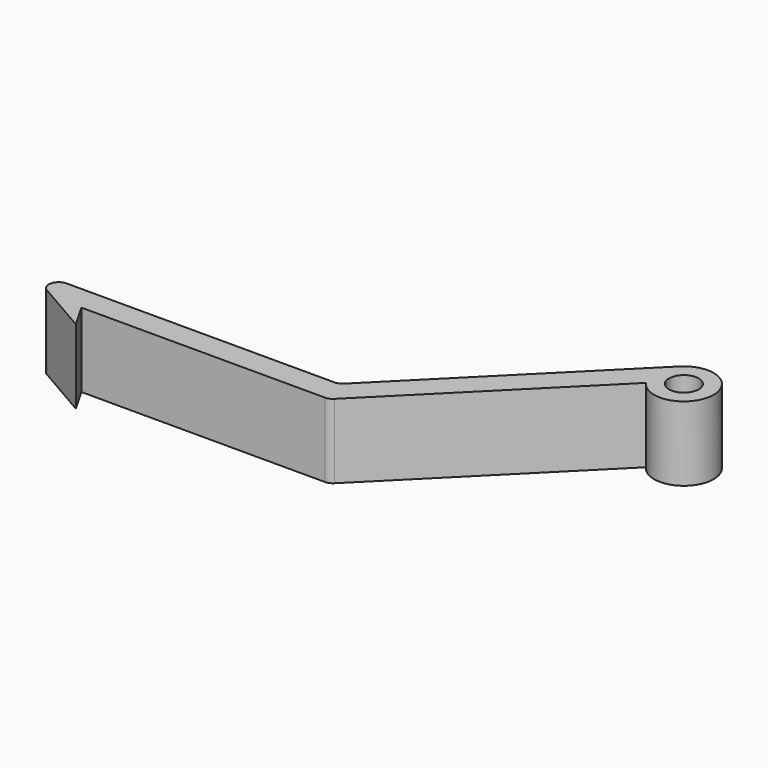
from build123d import *

# Parameters (mm, degrees)
F0_R     = 3
F1_DEPTH = 15
F2_W     = 7
F2_H     = 5
F3_DEPTH = 10
F4_F1_R  = 2
F4_F2_R  = 2
F5_R     = 2


with BuildPart() as f1:
    # F0 (on Top) → F1 (new body)
    with BuildSketch(Plane.XY):
        with BuildLine():
            Line((-40.4142135624, -39), (-4.8904069139, -3.4761933515))
            ThreePointArc((-4.8904069139, -3.4761933515), (5.9789831367, -0.5017575617), (-4.2426406871, 4.2426406871))
            Line((-4.2426406871, 4.2426406871), (-42.4852813742, -34))
            Line((-42.4852813742, -34), (-104.8479702921, -34))
            Line((-104.8479702921, -34), (-87.5274622164, -44))
            Line((-87.5274622164, -44), (-90.4142135624, -39))
            Line((-90.4142135624, -39), (-40.4142135624, -39))
        make_face()
        Circle(F0_R, mode=Mode.SUBTRACT)
    extrude(amount=F1_DEPTH)

    # F2 (on face) → F3 (join)
    with BuildSketch(Plane(origin=(-4.2426406871, 4.2426406871, 0), x_dir=(-0.7071067812, -0.7071067812, 0), z_dir=(-0.7071067812, 0.7071067812, 0))):
        with Locations((36.5832611207, 7.5)):
            Rectangle(F2_W, F2_H)
    extrude(amount=F3_DEPTH)

    # F4: fillet of radius 2 on 9 edges, made by hand

    # F4_f1
    f4_f1_edges = [f1.edges().sort_by_distance(p)[0] for p in [
        (-36.1213203436, -20.5649711575, 10),
        (-36.1213203436, -20.5649711575, 5),
        (-31.1715728753, -15.6152236891, 5),
        (-31.1715728753, -15.6152236891, 10),
        (-37.1819805153, -14.5545635174, 10),
        (-37.1819805153, -14.5545635174, 5),
        (-34.7071067812, -12.0796897832, 7.5),
        (-39.6568542495, -17.0294372515, 7.5),
    ]]
    fillet(f4_f1_edges, radius=F4_F1_R)

    # F4_f2
    f4_f2_edges = [f1.edges().sort_by_distance(p)[0] for p in [
        (-32.5857864376, -24.1005050634, 7.5),
        (-32.1715728753, -23.686291501, 5.5857864376),
        (-32.1715728753, -23.686291501, 9.4142135624),
    ]]
    fillet(f4_f2_edges, radius=F4_F2_R)

    # F5
    f5_edges = [f1.edges().sort_by_distance(p)[0] for p in [
        (-104.84797, -34, 7.5),
        (-40.414214, -39, 7.5),
        (-42.485281, -34, 7.5),
    ]]
    fillet(f5_edges, radius=F5_R)


solid = f1.part
